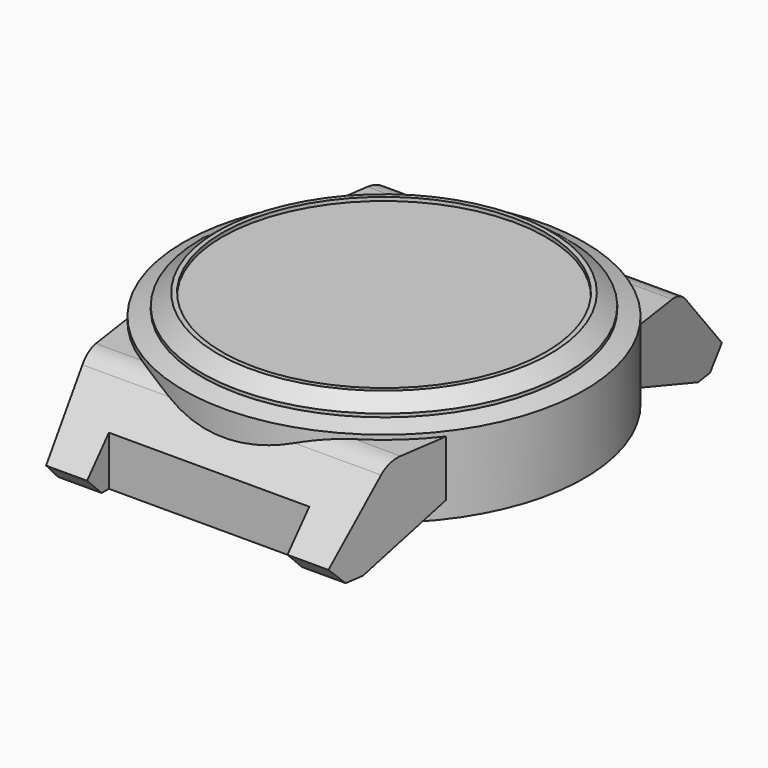
from build123d import *

# Parameters (mm, degrees)
F3_DEPTH         = 17.5
F5_DEPTH         = 12.801
F5_COPIES2_COUNT = 2
F6_W             = 22
F6_H             = 3
F7_DEPTH         = 12.801


# Not quite as in the source:
# - a pattern or mirror of a feature is missing from the dataset's text; its kind, count and spacing are read off the source's solid


with BuildPart() as f1:
    # F0 (on Front) → F1 (revolve)
    with BuildSketch(Plane.XZ):
        Polygon((-15, 0), (0, 0), (0, 12.4), (-17.75, 12.4), (-17.75, 12.8), (-18.25, 12.8), (-20, 11.5), (-20, 11.1382370815), (-22, 10.5), (-22, 2), (-19, 2), align=None)
    revolve(axis=Axis((0, 0, 3.4052523688), (0, 0, -1)))

    # F2 (on Right) → F3 (join, symmetric)
    with BuildSketch(Plane.YZ):
        with BuildLine():
            Line((23, 0), (25, 0))
            Line((25, 0), (27, 2))
            Line((27, 2), (20.8964254043, 8.9755138236))
            ThreePointArc((20.8964254043, 8.9755138236), (19.8783441675, 9.7318987418), (18.6386953202, 10))
            Line((18.6386953202, 10), (13, 10))
            Line((13, 10), (13, 4))
            Line((13, 4), (23, 0))
        make_face()
    f3 = extrude(amount=F3_DEPTH, both=True)

    # F3_copies: F3 across plane
    add(f3.mirror(Plane(origin=(0, 0, 0), x_dir=(0, 0, -1), z_dir=(0, -1, 0))))

    # F4 (on Top) → F5 (cut, through all)
    with BuildSketch(Plane.XY):
        Polygon((-17.5, 27), (-17.5, 13.332291626), (-15.5, 27), align=None)
    f5 = extrude(amount=F5_DEPTH, mode=Mode.SUBTRACT)

    # F5_copies: F5 across plane
    add(f5.mirror(Plane(origin=(0, 0, 0), x_dir=(0, 0, 1), z_dir=(1, 0, 0))), mode=Mode.SUBTRACT)

    # F5_copies1: F5 across plane
    add(f5.mirror(Plane(origin=(0, 0, 0), x_dir=(0, 0, -1), z_dir=(0, -1, 0))), mode=Mode.SUBTRACT)

    # F5_copies2: F5 ×2 about axis
    f5_copies2_axis = Axis((0, 0, 0), (0, 0, 1))
    for i in range(1, F5_COPIES2_COUNT):
        add(f5.rotate(f5_copies2_axis, i * 360 / F5_COPIES2_COUNT), mode=Mode.SUBTRACT)

    # F6 (on Top) → F7 (cut, through all)
    with BuildSketch(Plane.XY):
        with Locations((0, 25.5)):
            Rectangle(F6_W, F6_H)
    f7 = extrude(amount=F7_DEPTH, mode=Mode.SUBTRACT)

    # F7_copies: F7 across plane
    add(f7.mirror(Plane(origin=(0, 0, 0), x_dir=(0, 0, -1), z_dir=(0, -1, 0))), mode=Mode.SUBTRACT)


solid = f1.part
